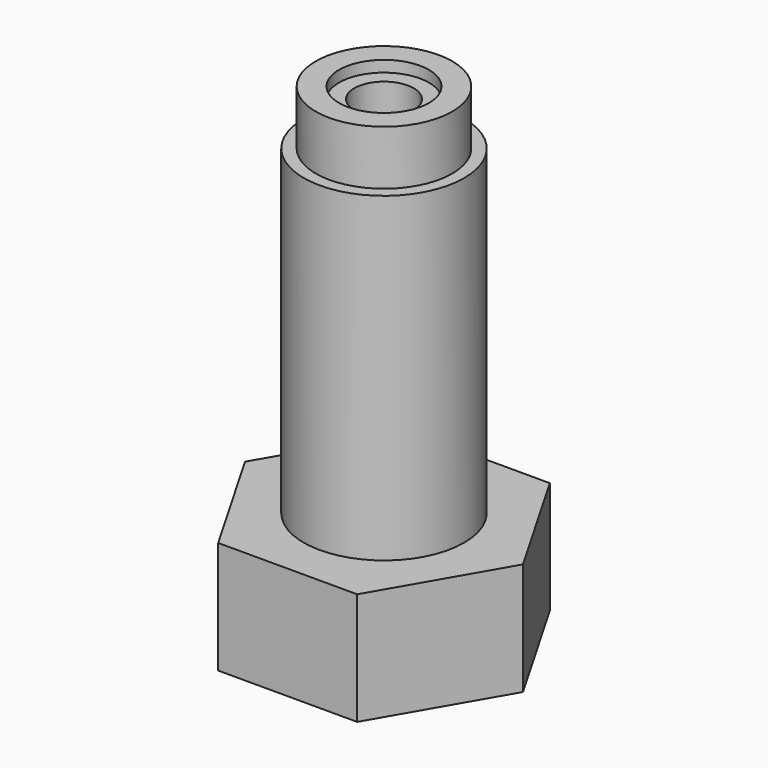
from build123d import *

# Parameters (mm, degrees)
F6_DEPTH  = 8.89
F7_R      = 6.35
F8_DEPTH  = 25.4
F9_R      = 5.3975
F10_DEPTH = 4.318
F11_R     = 3.556
F12_DEPTH = 0.889
F13_R     = 2.3495
F14_DEPTH = 9.7282


# Not quite as in the source:
# - a variable given as a bare number and used for a length is read in inches; the dataset says mm whatever the document's units were


with BuildPart() as f6:
    # F5 (on Top) → F6 (new body)
    with BuildSketch(Plane.XY):
        Polygon((5.499261314, 9.525), (-5.499261314, 9.525), (-10.9985226281, 0), (-5.499261314, -9.525), (5.499261314, -9.525), (10.9985226281, 0), align=None)
    extrude(amount=F6_DEPTH)

    # F7 (on face) → F8 (join)
    with BuildSketch(Plane.XY.offset(8.89)):
        Circle(F7_R)
    extrude(amount=F8_DEPTH)

    # F9 (on face) → F10 (join)
    with BuildSketch(Plane.XY.offset(34.29)):
        Circle(F9_R)
    extrude(amount=F10_DEPTH)

    # F11 (on face) → F12 (cut)
    with BuildSketch(Plane.XY.offset(38.608)):
        Circle(F11_R)
    extrude(amount=-F12_DEPTH, mode=Mode.SUBTRACT)

    # F13 (on face) → F14 (cut)
    with BuildSketch(Plane.XY.offset(38.608)):
        Circle(F13_R)
    extrude(amount=-F14_DEPTH, mode=Mode.SUBTRACT)


solid = f6.part
